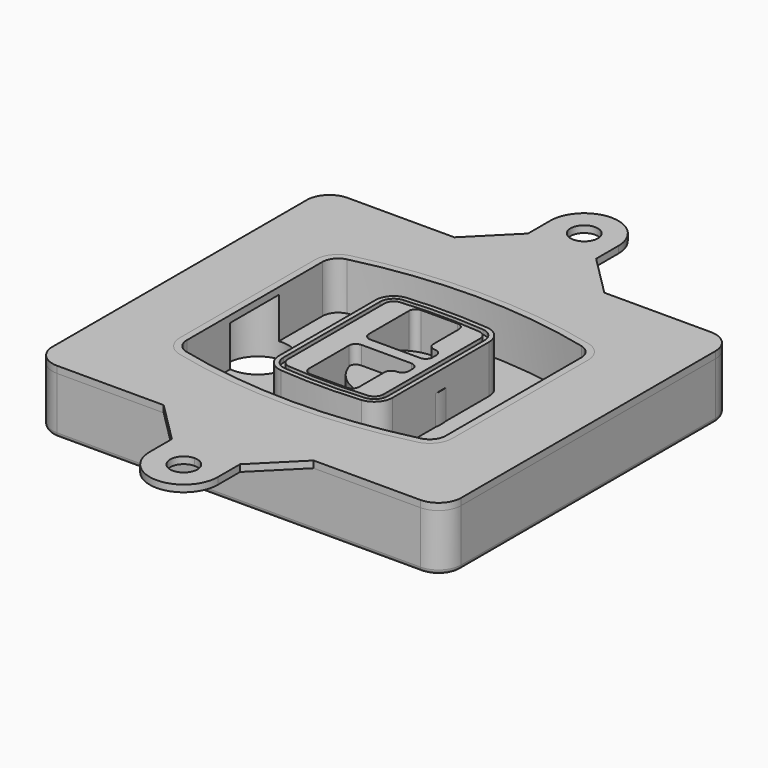
from build123d import *

# Parameters (mm, degrees)
F0_R      = 4
F1_DEPTH  = 25
F2_DEPTH  = 3
F3_DEPTH  = 18
F5_DEPTH  = 21
F6_DEPTH  = 2
F8_DEPTH  = 20
F9_DEPTH  = 16
F10_DEPTH = 25
F7_R      = 6
F7_R_2    = 4
F11_DEPTH = 6
F13_DEPTH = 9
F15_R     = 2
F17_DEPTH = 3


# Not quite as in the source:
# - a feature of the source that left no trace in its solid (it failed there, or was rolled back) is left out
# - a feature names something its author has since deleted; it is built from what else it names


with BuildPart() as f1:
    # F0 (on Top) → F1 (new body)
    with BuildSketch(Plane.XY):
        with BuildLine():
            ThreePointArc((-90, -70), (-87.0710678119, -77.0710678119), (-80, -80))
            Line((-80, -80), (80, -80))
            ThreePointArc((80, -80), (87.0710678119, -77.0710678119), (90, -70))
            Line((90, -70), (90, 70))
            ThreePointArc((90, 70), (87.0710678119, 77.0710678119), (80, 80))
            Line((80, 80), (-80, 80))
            ThreePointArc((-80, 80), (-87.0710678119, 77.0710678119), (-90, 70))
            Line((-90, 70), (-90, -70))
        make_face()
        with Locations((-60, -53.3333333333)):
            Circle(F0_R, mode=Mode.SUBTRACT)
        with Locations((60, -53.3333333333)):
            Circle(F0_R, mode=Mode.SUBTRACT)
        with Locations((-60, 53.3333333333)):
            Circle(F0_R, mode=Mode.SUBTRACT)
        with BuildLine():
            ThreePointArc((-64, 37.2990447398), (-61.0143011354, 45.9411029726), (-53.3306899286, 50.8970778549))
            ThreePointArc((-53.3306899286, 50.8970778549), (0, 57.3333333333), (53.3306899286, 50.8970778549))
            ThreePointArc((53.3306899286, 50.8970778549), (61.0143011354, 45.9411029726), (64, 37.2990447398))
            Line((64, 37.2990447398), (64, -37.2990447398))
            ThreePointArc((64, -37.2990447398), (61.0143011354, -45.9411029726), (53.3306899286, -50.8970778549))
            ThreePointArc((53.3306899286, -50.8970778549), (0, -57.3333333333), (-53.3306899286, -50.8970778549))
            ThreePointArc((-53.3306899286, -50.8970778549), (-61.0143011354, -45.9411029726), (-64, -37.2990447398))
            Line((-64, -37.2990447398), (-64, 37.2990447398))
        make_face(mode=Mode.SUBTRACT)
        with Locations((60, 53.3333333333)):
            Circle(F0_R, mode=Mode.SUBTRACT)
        with BuildLine():
            ThreePointArc((53.3306899286, 50.8970778549), (0, 57.3333333333), (-53.3306899286, 50.8970778549))
            ThreePointArc((-53.3306899286, 50.8970778549), (-61.0143011354, 45.9411029726), (-64, 37.2990447398))
            Line((-64, 37.2990447398), (-64, -37.2990447398))
            ThreePointArc((-64, -37.2990447398), (-61.0143011354, -45.9411029726), (-53.3306899286, -50.8970778549))
            ThreePointArc((-53.3306899286, -50.8970778549), (0, -57.3333333333), (53.3306899286, -50.8970778549))
            ThreePointArc((53.3306899286, -50.8970778549), (61.0143011354, -45.9411029726), (64, -37.2990447398))
            Line((64, -37.2990447398), (64, 37.2990447398))
            ThreePointArc((64, 37.2990447398), (61.0143011354, 45.9411029726), (53.3306899286, 50.8970778549))
        make_face()
        with BuildLine():
            Line((-60, -37.2990447398), (-60, 37.2990447398))
            ThreePointArc((-60, 37.2990447398), (-57.8673579538, 43.4719434775), (-52.3790642347, 47.0119255363))
            ThreePointArc((-52.3790642347, 47.0119255363), (0, 53.3333333333), (52.3790642347, 47.0119255363))
            ThreePointArc((52.3790642347, 47.0119255363), (57.8673579538, 43.4719434775), (60, 37.2990447398))
            Line((60, 37.2990447398), (60, -37.2990447398))
            ThreePointArc((60, -37.2990447398), (57.8673579538, -43.4719434775), (52.3790642347, -47.0119255363))
            ThreePointArc((52.3790642347, -47.0119255363), (0, -53.3333333333), (-52.3790642347, -47.0119255363))
            ThreePointArc((-52.3790642347, -47.0119255363), (-57.8673579538, -43.4719434775), (-60, -37.2990447398))
        make_face(mode=Mode.SUBTRACT)
        with BuildLine():
            ThreePointArc((-52.3790642347, 47.0119255363), (-57.8673579538, 43.4719434775), (-60, 37.2990447398))
            Line((-60, 37.2990447398), (-60, -37.2990447398))
            ThreePointArc((-60, -37.2990447398), (-57.8673579538, -43.4719434775), (-52.3790642347, -47.0119255363))
            ThreePointArc((-52.3790642347, -47.0119255363), (0, -53.3333333333), (52.3790642347, -47.0119255363))
            ThreePointArc((52.3790642347, -47.0119255363), (57.8673579538, -43.4719434775), (60, -37.2990447398))
            Line((60, -37.2990447398), (60, 37.2990447398))
            ThreePointArc((60, 37.2990447398), (57.8673579538, 43.4719434775), (52.3790642347, 47.0119255363))
            ThreePointArc((52.3790642347, 47.0119255363), (0, 53.3333333333), (-52.3790642347, 47.0119255363))
        make_face()
        with BuildLine():
            ThreePointArc((51.6653449643, 44.0980612973), (55.5071505677, 41.6200738562), (57, 37.2990447398))
            Line((57, 37.2990447398), (57, -37.2990447398))
            ThreePointArc((57, -37.2990447398), (55.5071505677, -41.6200738562), (51.6653449643, -44.0980612973))
            ThreePointArc((51.6653449643, -44.0980612973), (0, -50.3333333333), (-51.6653449643, -44.0980612973))
            ThreePointArc((-51.6653449643, -44.0980612973), (-55.5071505677, -41.6200738562), (-57, -37.2990447398))
            Line((-57, -37.2990447398), (-57, 37.2990447398))
            ThreePointArc((-57, 37.2990447398), (-55.5071505677, 41.6200738562), (-51.6653449643, 44.0980612973))
            ThreePointArc((-51.6653449643, 44.0980612973), (0, 50.3333333333), (51.6653449643, 44.0980612973))
        make_face(mode=Mode.SUBTRACT)
        with BuildLine():
            Line((57, -37.2990447398), (57, 37.2990447398))
            ThreePointArc((57, 37.2990447398), (55.5071505677, 41.6200738562), (51.6653449643, 44.0980612973))
            ThreePointArc((51.6653449643, 44.0980612973), (0, 50.3333333333), (-51.6653449643, 44.0980612973))
            ThreePointArc((-51.6653449643, 44.0980612973), (-55.5071505677, 41.6200738562), (-57, 37.2990447398))
            Line((-57, 37.2990447398), (-57, -37.2990447398))
            ThreePointArc((-57, -37.2990447398), (-55.5071505677, -41.6200738562), (-51.6653449643, -44.0980612973))
            ThreePointArc((-51.6653449643, -44.0980612973), (0, -50.3333333333), (51.6653449643, -44.0980612973))
            ThreePointArc((51.6653449643, -44.0980612973), (55.5071505677, -41.6200738562), (57, -37.2990447398))
        make_face()
    extrude(amount=-F1_DEPTH)

    # F0 (on Top) → F2 (join)
    with BuildSketch(Plane.XY):
        with BuildLine():
            ThreePointArc((-52.3790642347, 47.0119255363), (-57.8673579538, 43.4719434775), (-60, 37.2990447398))
            Line((-60, 37.2990447398), (-60, -37.2990447398))
            ThreePointArc((-60, -37.2990447398), (-57.8673579538, -43.4719434775), (-52.3790642347, -47.0119255363))
            ThreePointArc((-52.3790642347, -47.0119255363), (0, -53.3333333333), (52.3790642347, -47.0119255363))
            ThreePointArc((52.3790642347, -47.0119255363), (57.8673579538, -43.4719434775), (60, -37.2990447398))
            Line((60, -37.2990447398), (60, 37.2990447398))
            ThreePointArc((60, 37.2990447398), (57.8673579538, 43.4719434775), (52.3790642347, 47.0119255363))
            ThreePointArc((52.3790642347, 47.0119255363), (0, 53.3333333333), (-52.3790642347, 47.0119255363))
        make_face()
        with BuildLine():
            ThreePointArc((51.6653449643, 44.0980612973), (55.5071505677, 41.6200738562), (57, 37.2990447398))
            Line((57, 37.2990447398), (57, -37.2990447398))
            ThreePointArc((57, -37.2990447398), (55.5071505677, -41.6200738562), (51.6653449643, -44.0980612973))
            ThreePointArc((51.6653449643, -44.0980612973), (0, -50.3333333333), (-51.6653449643, -44.0980612973))
            ThreePointArc((-51.6653449643, -44.0980612973), (-55.5071505677, -41.6200738562), (-57, -37.2990447398))
            Line((-57, -37.2990447398), (-57, 37.2990447398))
            ThreePointArc((-57, 37.2990447398), (-55.5071505677, 41.6200738562), (-51.6653449643, 44.0980612973))
            ThreePointArc((-51.6653449643, 44.0980612973), (0, 50.3333333333), (51.6653449643, 44.0980612973))
        make_face(mode=Mode.SUBTRACT)
    extrude(amount=F2_DEPTH)

    # F0 (on Top) → F3 (cut)
    with BuildSketch(Plane.XY):
        with BuildLine():
            Line((57, -37.2990447398), (57, 37.2990447398))
            ThreePointArc((57, 37.2990447398), (55.5071505677, 41.6200738562), (51.6653449643, 44.0980612973))
            ThreePointArc((51.6653449643, 44.0980612973), (0, 50.3333333333), (-51.6653449643, 44.0980612973))
            ThreePointArc((-51.6653449643, 44.0980612973), (-55.5071505677, 41.6200738562), (-57, 37.2990447398))
            Line((-57, 37.2990447398), (-57, -37.2990447398))
            ThreePointArc((-57, -37.2990447398), (-55.5071505677, -41.6200738562), (-51.6653449643, -44.0980612973))
            ThreePointArc((-51.6653449643, -44.0980612973), (0, -50.3333333333), (51.6653449643, -44.0980612973))
            ThreePointArc((51.6653449643, -44.0980612973), (55.5071505677, -41.6200738562), (57, -37.2990447398))
        make_face()
    extrude(amount=-F3_DEPTH, mode=Mode.SUBTRACT)

    # F4 (on face) → F5 (join, through all)
    with BuildSketch(Plane.XY.offset(3)):
        with BuildLine():
            ThreePointArc((-25, -26.587695628), (-22.8992979869, -31.9912392117), (-17.7004291845, -34.5569740744))
            ThreePointArc((-17.7004291845, -34.5569740744), (0, -35.3333333333), (17.7004291845, -34.5569740744))
            ThreePointArc((17.7004291845, -34.5569740744), (22.8992979869, -31.9912392117), (25, -26.587695628))
            Line((25, -26.587695628), (25, 26.587695628))
            ThreePointArc((25, 26.587695628), (22.8992979869, 31.9912392117), (17.7004291845, 34.5569740744))
            ThreePointArc((17.7004291845, 34.5569740744), (0, 35.3333333333), (-17.7004291845, 34.5569740744))
            ThreePointArc((-17.7004291845, 34.5569740744), (-22.8992979869, 31.9912392117), (-25, 26.587695628))
            Line((-25, 26.587695628), (-25, -26.587695628))
        make_face()
        with BuildLine():
            ThreePointArc((17.5253218884, 32.5646544628), (21.4244734902, 30.6403533158), (23, 26.587695628))
            Line((23, 26.587695628), (23, -26.587695628))
            ThreePointArc((23, -26.587695628), (21.4244734902, -30.6403533158), (17.5253218884, -32.5646544628))
            ThreePointArc((17.5253218884, -32.5646544628), (0, -33.3333333333), (-17.5253218884, -32.5646544628))
            ThreePointArc((-17.5253218884, -32.5646544628), (-21.4244734902, -30.6403533158), (-23, -26.587695628))
            Line((-23, -26.587695628), (-23, 26.587695628))
            ThreePointArc((-23, 26.587695628), (-21.4244734902, 30.6403533158), (-17.5253218884, 32.5646544628))
            ThreePointArc((-17.5253218884, 32.5646544628), (0, 33.3333333333), (17.5253218884, 32.5646544628))
        make_face(mode=Mode.SUBTRACT)
        with BuildLine():
            Line((23, -26.587695628), (23, 26.587695628))
            ThreePointArc((23, 26.587695628), (21.4244734902, 30.6403533158), (17.5253218884, 32.5646544628))
            ThreePointArc((17.5253218884, 32.5646544628), (0, 33.3333333333), (-17.5253218884, 32.5646544628))
            ThreePointArc((-17.5253218884, 32.5646544628), (-21.4244734902, 30.6403533158), (-23, 26.587695628))
            Line((-23, 26.587695628), (-23, -26.587695628))
            ThreePointArc((-23, -26.587695628), (-21.4244734902, -30.6403533158), (-17.5253218884, -32.5646544628))
            ThreePointArc((-17.5253218884, -32.5646544628), (0, -33.3333333333), (17.5253218884, -32.5646544628))
            ThreePointArc((17.5253218884, -32.5646544628), (21.4244734902, -30.6403533158), (23, -26.587695628))
        make_face()
        with BuildLine():
            ThreePointArc((17.3502145923, 30.5723348512), (19.9496489934, 29.2894674198), (21, 26.587695628))
            Line((21, 26.587695628), (21, -26.587695628))
            ThreePointArc((21, -26.587695628), (19.9496489934, -29.2894674198), (17.3502145923, -30.5723348512))
            ThreePointArc((17.3502145923, -30.5723348512), (0, -31.3333333333), (-17.3502145923, -30.5723348512))
            ThreePointArc((-17.3502145923, -30.5723348512), (-19.9496489934, -29.2894674198), (-21, -26.587695628))
            Line((-21, -26.587695628), (-21, 26.587695628))
            ThreePointArc((-21, 26.587695628), (-19.9496489934, 29.2894674198), (-17.3502145923, 30.5723348512))
            ThreePointArc((-17.3502145923, 30.5723348512), (0, 31.3333333333), (17.3502145923, 30.5723348512))
        make_face(mode=Mode.SUBTRACT)
        with BuildLine():
            Line((21, -26.587695628), (21, 26.587695628))
            ThreePointArc((21, 26.587695628), (19.9496489934, 29.2894674198), (17.3502145923, 30.5723348512))
            ThreePointArc((17.3502145923, 30.5723348512), (0, 31.3333333333), (-17.3502145923, 30.5723348512))
            ThreePointArc((-17.3502145923, 30.5723348512), (-19.9496489934, 29.2894674198), (-21, 26.587695628))
            Line((-21, 26.587695628), (-21, -26.587695628))
            ThreePointArc((-21, -26.587695628), (-19.9496489934, -29.2894674198), (-17.3502145923, -30.5723348512))
            ThreePointArc((-17.3502145923, -30.5723348512), (0, -31.3333333333), (17.3502145923, -30.5723348512))
            ThreePointArc((17.3502145923, -30.5723348512), (19.9496489934, -29.2894674198), (21, -26.587695628))
        make_face()
        with BuildLine():
            Line((-8, -2.5), (14, -2.5))
            ThreePointArc((14, -2.5), (16.1213203436, -3.3786796564), (17, -5.5))
            Line((17, -5.5), (17, -7.5))
            ThreePointArc((17, -7.5), (16.1213203436, -9.6213203436), (14, -10.5))
            ThreePointArc((14, -10.5), (11.8786796564, -11.3786796564), (11, -13.5))
            Line((11, -13.5), (11, -27.5))
            ThreePointArc((11, -27.5), (10.1213203436, -29.6213203436), (8, -30.5))
            Line((8, -30.5), (-8, -30.5))
            ThreePointArc((-8, -30.5), (-10.1213203436, -29.6213203436), (-11, -27.5))
            Line((-11, -27.5), (-11, -5.5))
            ThreePointArc((-11, -5.5), (-10.1213203436, -3.3786796564), (-8, -2.5))
        make_face(mode=Mode.SUBTRACT)
        with BuildLine():
            ThreePointArc((-8, 2.5), (-10.1213203436, 3.3786796564), (-11, 5.5))
            Line((-11, 5.5), (-11, 27.5))
            ThreePointArc((-11, 27.5), (-10.1213203436, 29.6213203436), (-8, 30.5))
            Line((-8, 30.5), (8, 30.5))
            ThreePointArc((8, 30.5), (10.1213203436, 29.6213203436), (11, 27.5))
            Line((11, 27.5), (11, 13.5))
            ThreePointArc((11, 13.5), (11.8786796564, 11.3786796564), (14, 10.5))
            ThreePointArc((14, 10.5), (16.1213203436, 9.6213203436), (17, 7.5))
            Line((17, 7.5), (17, 5.5))
            ThreePointArc((17, 5.5), (16.1213203436, 3.3786796564), (14, 2.5))
            Line((14, 2.5), (-8, 2.5))
        make_face(mode=Mode.SUBTRACT)
    extrude(amount=-F5_DEPTH)

    # F4 (on face) → F6 (cut)
    with BuildSketch(Plane.XY.offset(3)):
        with BuildLine():
            Line((23, -26.587695628), (23, 26.587695628))
            ThreePointArc((23, 26.587695628), (21.4244734902, 30.6403533158), (17.5253218884, 32.5646544628))
            ThreePointArc((17.5253218884, 32.5646544628), (0, 33.3333333333), (-17.5253218884, 32.5646544628))
            ThreePointArc((-17.5253218884, 32.5646544628), (-21.4244734902, 30.6403533158), (-23, 26.587695628))
            Line((-23, 26.587695628), (-23, -26.587695628))
            ThreePointArc((-23, -26.587695628), (-21.4244734902, -30.6403533158), (-17.5253218884, -32.5646544628))
            ThreePointArc((-17.5253218884, -32.5646544628), (0, -33.3333333333), (17.5253218884, -32.5646544628))
            ThreePointArc((17.5253218884, -32.5646544628), (21.4244734902, -30.6403533158), (23, -26.587695628))
        make_face()
        with BuildLine():
            ThreePointArc((17.3502145923, 30.5723348512), (19.9496489934, 29.2894674198), (21, 26.587695628))
            Line((21, 26.587695628), (21, -26.587695628))
            ThreePointArc((21, -26.587695628), (19.9496489934, -29.2894674198), (17.3502145923, -30.5723348512))
            ThreePointArc((17.3502145923, -30.5723348512), (0, -31.3333333333), (-17.3502145923, -30.5723348512))
            ThreePointArc((-17.3502145923, -30.5723348512), (-19.9496489934, -29.2894674198), (-21, -26.587695628))
            Line((-21, -26.587695628), (-21, 26.587695628))
            ThreePointArc((-21, 26.587695628), (-19.9496489934, 29.2894674198), (-17.3502145923, 30.5723348512))
            ThreePointArc((-17.3502145923, 30.5723348512), (0, 31.3333333333), (17.3502145923, 30.5723348512))
        make_face(mode=Mode.SUBTRACT)
    extrude(amount=-F6_DEPTH, mode=Mode.SUBTRACT)

    # F7 (on face) → F8 (join)
    with BuildSketch(Plane(origin=(0, 0, -25), x_dir=(1, 0, 0), z_dir=(0, 0, -1))):
        with BuildLine():
            ThreePointArc((-6.71157564, 0), (6.7567035675, 13.4682792075), (20.224982775, 0))
            Line((20.224982775, 0), (25.224982775, 0))
            ThreePointArc((25.224982775, 0), (6.7567035675, 18.4682792075), (-11.71157564, 0))
            Line((-11.71157564, 0), (-6.71157564, 0))
        make_face()
        with BuildLine():
            Line((-6.71157564, 0), (20.224982775, 0))
            ThreePointArc((20.224982775, 0), (6.7567035675, 13.4682792075), (-6.71157564, 0))
        make_face()
        with BuildLine():
            ThreePointArc((-6.71157564, 0), (6.7567035675, -13.4682792075), (20.224982775, 0))
            Line((20.224982775, 0), (-6.71157564, 0))
        make_face()
        with BuildLine():
            Line((25.224982775, 0), (20.224982775, 0))
            ThreePointArc((20.224982775, 0), (6.7567035675, -13.4682792075), (-6.71157564, 0))
            Line((-6.71157564, 0), (-11.71157564, 0))
            ThreePointArc((-11.71157564, 0), (6.7567035675, -18.4682792075), (25.224982775, 0))
        make_face()
    extrude(amount=-F8_DEPTH)

    # F7 (on face) → F9 (cut)
    with BuildSketch(Plane(origin=(0, 0, -25), x_dir=(1, 0, 0), z_dir=(0, 0, -1))):
        with BuildLine():
            Line((-6.71157564, 0), (20.224982775, 0))
            ThreePointArc((20.224982775, 0), (6.7567035675, 13.4682792075), (-6.71157564, 0))
        make_face()
        with BuildLine():
            ThreePointArc((-6.71157564, 0), (6.7567035675, -13.4682792075), (20.224982775, 0))
            Line((20.224982775, 0), (-6.71157564, 0))
        make_face()
    extrude(amount=-F9_DEPTH, mode=Mode.SUBTRACT)

    # F7 (on face) → F10 (cut)
    with BuildSketch(Plane(origin=(0, 0, -25), x_dir=(1, 0, 0), z_dir=(0, 0, -1))):
        with BuildLine():
            Line((-69.0318229325, 0), (-42.0952645175, 0))
            ThreePointArc((-42.0952645175, 0), (-55.563543725, 13.4682792075), (-69.0318229325, 0))
        make_face()
        with BuildLine():
            ThreePointArc((-69.0318229325, 0), (-55.563543725, -13.4682792075), (-42.0952645175, 0))
            Line((-42.0952645175, 0), (-69.0318229325, 0))
        make_face()
    extrude(amount=-F10_DEPTH, mode=Mode.SUBTRACT)

    # F7 (on face) → F11 (cut)
    with BuildSketch(Plane(origin=(0, 0, -25), x_dir=(1, 0, 0), z_dir=(0, 0, -1))):
        with Locations((60, -53.3333333333)):
            Circle(F7_R)
        with Locations((60, -53.3333333333)):
            Circle(F7_R_2, mode=Mode.SUBTRACT)
        with Locations((-60, -53.3333333333)):
            Circle(F7_R)
        with Locations((-60, -53.3333333333)):
            Circle(F7_R_2, mode=Mode.SUBTRACT)
        with Locations((-60, 53.3333333333)):
            Circle(F7_R)
        with Locations((-60, 53.3333333333)):
            Circle(F7_R_2, mode=Mode.SUBTRACT)
        with Locations((60, 53.3333333333)):
            Circle(F7_R)
        with Locations((60, 53.3333333333)):
            Circle(F7_R_2, mode=Mode.SUBTRACT)
    extrude(amount=-F11_DEPTH, mode=Mode.SUBTRACT)

    # F12 (on face) → F13 (cut, through all)
    with BuildSketch(Plane(origin=(0, 0, -9), x_dir=(1, 0, 0), z_dir=(0, 0, -1))):
        with BuildLine():
            ThreePointArc((20.224982775, 0), (20.1663399806, 1.2554664788), (19.9909222755, 2.5))
            Line((19.9909222755, 2.5), (14, 2.5))
            ThreePointArc((14, 2.5), (16.1213203436, 3.3786796564), (17, 5.5))
            Line((17, 5.5), (17, 7.5))
            ThreePointArc((17, 7.5), (16.1213203436, 9.6213203436), (14, 10.5))
            ThreePointArc((14, 10.5), (12.1627255951, 11.1284134507), (11.0951631559, 12.750384826))
            ThreePointArc((11.0951631559, 12.750384826), (11.0476113807, 12.7664660322), (11, 12.7823698976))
            Line((11, 12.7823698976), (11, -12.7823698976))
            ThreePointArc((11, -12.7823698976), (11.0476113807, -12.7664660322), (11.0951631559, -12.750384826))
            ThreePointArc((11.0951631559, -12.750384826), (12.1627255951, -11.1284134507), (14, -10.5))
            ThreePointArc((14, -10.5), (16.1213203436, -9.6213203436), (17, -7.5))
            Line((17, -7.5), (17, -5.5))
            ThreePointArc((17, -5.5), (16.1213203436, -3.3786796564), (14, -2.5))
            Line((14, -2.5), (19.9909222755, -2.5))
            ThreePointArc((19.9909222755, -2.5), (20.1663399806, -1.2554664788), (20.224982775, 0))
        make_face()
    extrude(amount=F13_DEPTH, mode=Mode.SUBTRACT)

    # F15
    f15_edges = [f1.edges().sort_by_distance(p)[0] for p in [
        (0, -80, -25),
        (-87.071068, -77.071068, -25),
        (-90, 0, -25),
        (-87.071068, 77.071068, -25),
        (87.071068, -77.071068, -25),
        (0, 80, -25),
        (90, 0, -25),
        (87.071068, 77.071068, -25),
    ]]
    fillet(f15_edges, radius=F15_R)


with BuildPart() as f17:
    # F16 (on face) → F17 (new body, through all)
    with BuildSketch(Plane.XY):
        with BuildLine():
            Line((-32.9987935502, 80), (-80, 80))
            ThreePointArc((-80, 80), (-87.0710678119, 77.0710678119), (-90, 70))
            Line((-90, 70), (-90, -70))
            ThreePointArc((-90, -70), (-87.0710678119, -77.0710678119), (-80, -80))
            Line((-80, -80), (-32.9987935502, -80))
            Line((-32.9987935502, -80), (0, -80))
            Line((0, -80), (33, -80))
            Line((33, -80), (80, -80))
            ThreePointArc((80, -80), (87.0710678119, -77.0710678119), (90, -70))
            Line((90, -70), (90, 70))
            ThreePointArc((90, 70), (87.0710678119, 77.0710678119), (80, 80))
            Line((80, 80), (33, 80))
            Line((33, 80), (0, 80))
            Line((0, 80), (-32.9987935502, 80))
        make_face()
        with BuildLine():
            ThreePointArc((-52.3790642347, 47.0119255363), (0, 53.3333333333), (52.3790642347, 47.0119255363))
            ThreePointArc((52.3790642347, 47.0119255363), (57.8673579538, 43.4719434775), (60, 37.2990447398))
            Line((60, 37.2990447398), (60, -37.2990447398))
            ThreePointArc((60, -37.2990447398), (57.8673579538, -43.4719434775), (52.3790642347, -47.0119255363))
            ThreePointArc((52.3790642347, -47.0119255363), (0, -53.3333333333), (-52.3790642347, -47.0119255363))
            ThreePointArc((-52.3790642347, -47.0119255363), (-57.8673579538, -43.4719434775), (-60, -37.2990447398))
            Line((-60, -37.2990447398), (-60, 37.2990447398))
            ThreePointArc((-60, 37.2990447398), (-57.8673579538, 43.4719434775), (-52.3790642347, 47.0119255363))
        make_face(mode=Mode.SUBTRACT)
        with BuildLine():
            Line((-14.9987935502, 98), (-32.9987935502, 80))
            Line((-32.9987935502, 80), (0, 80))
            Line((0, 80), (33, 80))
            Line((33, 80), (15, 98))
            Line((15, 98), (15, 110.1902420521))
            ThreePointArc((15, 110.1902420521), (-0.0951229387, 125.1899404366), (-14.9987935502, 110))
            Line((-14.9987935502, 110), (-14.9987935502, 98))
        make_face()
        with BuildLine():
            ThreePointArc((6, 110.1902420521), (4.2426406871, 105.947601365), (0, 104.1902420521))
            ThreePointArc((0, 104.1902420521), (-4.2426406871, 114.4328827392), (6, 110.1902420521))
        make_face(mode=Mode.SUBTRACT)
        with BuildLine():
            Line((0, -80), (-32.9987935502, -80))
            Line((-32.9987935502, -80), (-14.9987935502, -98))
            Line((-14.9987935502, -98), (-14.9987935502, -110))
            ThreePointArc((-14.9987935502, -110), (-0.0951229387, -125.1899404366), (15, -110.1902420521))
            Line((15, -110.1902420521), (15, -98))
            Line((15, -98), (33, -80))
            Line((33, -80), (0, -80))
        make_face()
        with BuildLine():
            ThreePointArc((6, -110.1902420521), (-4.2426406871, -114.4328827392), (0, -104.1902420521))
            ThreePointArc((0, -104.1902420521), (4.2426406871, -105.947601365), (6, -110.1902420521))
        make_face(mode=Mode.SUBTRACT)
    extrude(amount=F17_DEPTH)


solid = Compound([f1.part, f17.part])
